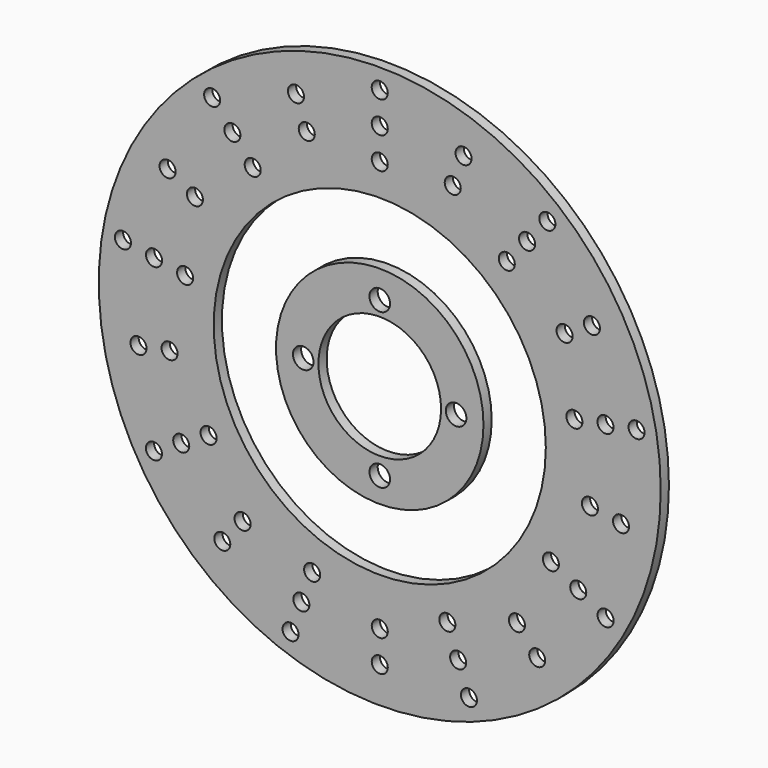
from build123d import *

# Parameters (mm, degrees)
F0_R            = 138.811
F0_R_2          = 82.042
F3_DEPTH        = 5.08
F2_R            = 3.9624
F4_DEPTH        = 5.081
F4_COPIES_COUNT = 9
F6_D            = 7.9248
F6_COPIES_COUNT = 9
F0_R_3          = 51.2445
F0_R_4          = 30.2895
F7_DEPTH        = 5.08
F8_D            = 10.16


# Not quite as in the source:
# - a pattern or mirror of a feature is missing from the dataset's text; its kind, count and spacing are read off the source's solid


with BuildPart() as f3:
    # F0 (on Front) → F3 (new body)
    with BuildSketch(Plane.XZ):
        Circle(F0_R)
        Circle(F0_R_2, mode=Mode.SUBTRACT)
    extrude(amount=F3_DEPTH)

    # F2 (on face) → F4 (cut, through all)
    with BuildSketch(Plane.XZ):
        with Locations((0, 97.6376)):
            Circle(F2_R)
        with Locations((0, 113.2332)):
            Circle(F2_R)
        with Locations((0, 128.8288)):
            Circle(F2_R)
    f4 = extrude(amount=F4_DEPTH, mode=Mode.SUBTRACT)

    # F4_copies: F4 ×9 about axis
    f4_copies_axis = Axis((0, 0, 0), (0, 1, 0))
    for i in range(1, F4_COPIES_COUNT):
        add(f4.rotate(f4_copies_axis, i * 360 / F4_COPIES_COUNT), mode=Mode.SUBTRACT)

    # F6 (through all)
    with Locations(Plane(origin=(0, 0, 0), x_dir=(1, 0, 0), z_dir=(0, 1, 0))):
        with Locations((0, 105.4354), (0, 121.031)):
            f6 = Hole(F6_D / 2)

    # F6_copies: F6 ×9 about axis
    f6_copies_axis = Axis((0, 0, 0), (0, 1, 0))
    for i in range(1, F6_COPIES_COUNT):
        add(f6.rotate(f6_copies_axis, i * 360 / F6_COPIES_COUNT), mode=Mode.SUBTRACT)


with BuildPart() as f7:
    # F0 (on Front) → F7 (new body)
    with BuildSketch(Plane.XZ):
        Circle(F0_R_3)
        Circle(F0_R_4, mode=Mode.SUBTRACT)
    extrude(amount=F7_DEPTH)

    # F8 (through all)
    with Locations(Plane(origin=(0, 0, 0), x_dir=(1, 0, 0), z_dir=(0, 1, 0))):
        with Locations((0, -37.5412), (37.7119863628, 0), (0, 38.8407654956), (-37.8069085799, 0)):
            Hole(F8_D / 2)


solid = Compound([f3.part, f7.part])
